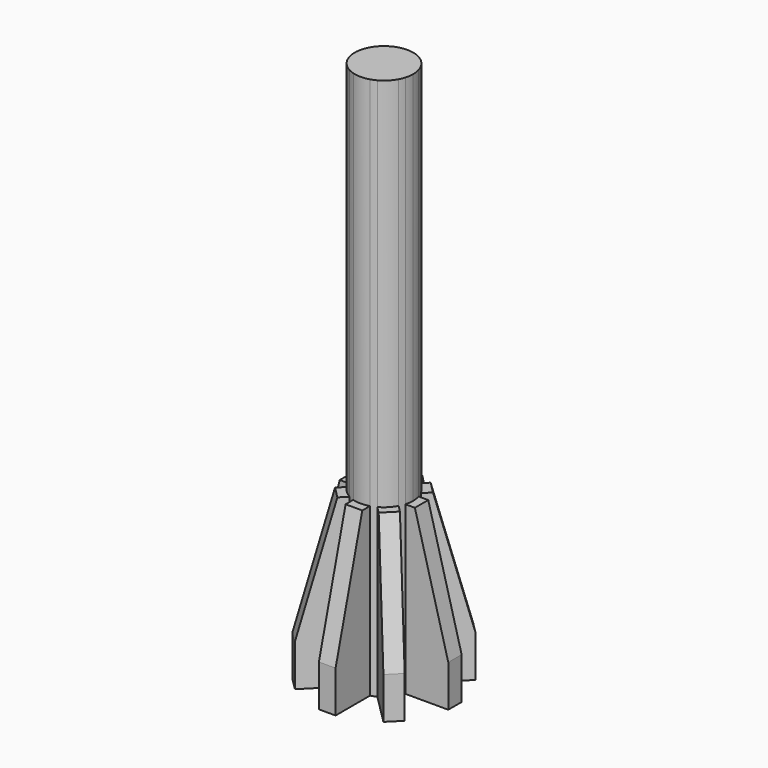
from build123d import *

# Parameters (mm, degrees)
F1_DEPTH   = 65
F2_DEPTH   = 20
F3_SIZE2   = 15
F3_SIZE    = 4
F3_2_SIZE2 = 15
F3_2_SIZE  = 4
F3_3_SIZE2 = 15
F3_3_SIZE  = 4
F3_4_SIZE2 = 15
F3_4_SIZE  = 4
F4_SIZE2   = 4
F4_SIZE    = 15
F4_2_SIZE2 = 4
F4_2_SIZE  = 15
F4_3_SIZE2 = 4
F4_3_SIZE  = 15
F4_4_SIZE2 = 4
F4_4_SIZE  = 15


with BuildPart() as f1:
    # F0 (on Top) → F1 (new body)
    with BuildSketch(Plane.XY):
        with BuildLine():
            Line((0.4761658125, 5.9305784088), (1.1407672764, 6.5951798727))
            ThreePointArc((1.1407672764, 6.5951798727), (0.8155578257, 6.7499432102), (0.4761658125, 6.8704668126))
            Line((0.4761658125, 6.8704668126), (0.4761658125, 5.9305784088))
        make_face()
        with BuildLine():
            Line((-3.6026492139, 1.8517633824), (-2.9380477499, 2.5163648464))
            Line((-2.9380477499, 2.5163648464), (-3.8779361538, 2.5163648464))
            ThreePointArc((-3.8779361538, 2.5163648464), (-3.7574125513, 2.1769728331), (-3.6026492139, 1.8517633824))
        make_face()
        with BuildLine():
            ThreePointArc((2.8302677787, 4.5163648464), (2.7097441763, 4.8557568597), (2.5549808388, 5.1809663103))
            Line((2.5549808388, 5.1809663103), (1.8903793748, 4.5163648464))
            Line((1.8903793748, 4.5163648464), (2.8302677787, 4.5163648464))
        make_face()
        with BuildLine():
            Line((-1.5238341875, 0.1622628801), (-1.5238341875, 1.102151284))
            Line((-1.5238341875, 1.102151284), (-2.1884356515, 0.4375498201))
            ThreePointArc((-2.1884356515, 0.4375498201), (-1.8632262008, 0.2827864826), (-1.5238341875, 0.1622628801))
        make_face()
        with BuildLine():
            ThreePointArc((2.5549808388, 5.1809663103), (1.9510395466, 5.9912385805), (1.1407672764, 6.5951798727))
            Line((1.1407672764, 6.5951798727), (0.4761658125, 5.9305784088))
            Line((0.4761658125, 5.9305784088), (0.4761658125, 4.5163648464))
            Line((0.4761658125, 4.5163648464), (1.8903793748, 4.5163648464))
            Line((1.8903793748, 4.5163648464), (2.5549808388, 5.1809663103))
        make_face()
        Polygon((-0.9380477499, 4.5163648464), (-0.5238341875, 4.9305784088), (-1.5238341875, 5.9305784088), (-1.5238341875, 4.5163648464), align=None)
        with BuildLine():
            Line((-1.5238341875, 2.5163648464), (-2.9380477499, 2.5163648464))
            Line((-2.9380477499, 2.5163648464), (-3.6026492139, 1.8517633824))
            ThreePointArc((-3.6026492139, 1.8517633824), (-2.9987079217, 1.0414911122), (-2.1884356515, 0.4375498201))
            Line((-2.1884356515, 0.4375498201), (-1.5238341875, 1.102151284))
            Line((-1.5238341875, 1.102151284), (-1.5238341875, 2.5163648464))
        make_face()
        Polygon((1.8903793748, 2.5163648464), (0.8903793748, 3.5163648464), (0.4761658125, 3.102151284), (0.4761658125, 2.5163648464), align=None)
        Polygon((-0.1096206252, 4.5163648464), (-0.5238341875, 4.9305784088), (-0.9380477499, 4.5163648464), align=None)
        with BuildLine():
            Line((-1.5238341875, 4.5163648464), (-1.5238341875, 5.9305784088))
            Line((-1.5238341875, 5.9305784088), (-2.1884356515, 6.5951798727))
            ThreePointArc((-2.1884356515, 6.5951798727), (-2.9987079217, 5.9912385805), (-3.6026492139, 5.1809663103))
            Line((-3.6026492139, 5.1809663103), (-2.9380477499, 4.5163648464))
            Line((-2.9380477499, 4.5163648464), (-1.5238341875, 4.5163648464))
        make_face()
        Polygon((0.4761658125, 2.5163648464), (0.4761658125, 3.102151284), (-0.1096206252, 2.5163648464), align=None)
        with BuildLine():
            Line((-2.9380477499, 2.5163648464), (-1.9380477499, 3.5163648464))
            Line((-1.9380477499, 3.5163648464), (-2.9380477499, 4.5163648464))
            Line((-2.9380477499, 4.5163648464), (-3.8779361538, 4.5163648464))
            ThreePointArc((-3.8779361538, 4.5163648464), (-4.0238341875, 3.5163648464), (-3.8779361538, 2.5163648464))
            Line((-3.8779361538, 2.5163648464), (-2.9380477499, 2.5163648464))
        make_face()
        with BuildLine():
            Line((-0.5238341875, 4.9305784088), (0.4761658125, 5.9305784088))
            Line((0.4761658125, 5.9305784088), (0.4761658125, 6.8704668126))
            ThreePointArc((0.4761658125, 6.8704668126), (-0.5238341875, 7.0163648464), (-1.5238341875, 6.8704668126))
            Line((-1.5238341875, 6.8704668126), (-1.5238341875, 5.9305784088))
            Line((-1.5238341875, 5.9305784088), (-0.5238341875, 4.9305784088))
        make_face()
        with BuildLine():
            Line((2.8302677787, 4.5163648464), (1.8903793748, 4.5163648464))
            Line((1.8903793748, 4.5163648464), (0.8903793748, 3.5163648464))
            Line((0.8903793748, 3.5163648464), (1.8903793748, 2.5163648464))
            Line((1.8903793748, 2.5163648464), (2.8302677787, 2.5163648464))
            ThreePointArc((2.8302677787, 2.5163648464), (2.9394992415, 3.0110713089), (2.9761658125, 3.5163648464))
            ThreePointArc((2.9761658125, 3.5163648464), (2.9394992415, 4.0216583839), (2.8302677787, 4.5163648464))
        make_face()
        Polygon((-1.5238341875, 3.102151284), (-1.5238341875, 3.9305784088), (-1.9380477499, 3.5163648464), align=None)
        Polygon((0.4761658125, 4.5163648464), (0.4761658125, 5.9305784088), (-0.5238341875, 4.9305784088), (-0.1096206252, 4.5163648464), align=None)
        Polygon((-1.5238341875, 3.9305784088), (-0.9380477499, 4.5163648464), (-1.5238341875, 4.5163648464), align=None)
        with BuildLine():
            Line((2.5549808388, 1.8517633824), (1.8903793748, 2.5163648464))
            Line((1.8903793748, 2.5163648464), (0.4761658125, 2.5163648464))
            Line((0.4761658125, 2.5163648464), (0.4761658125, 1.102151284))
            Line((0.4761658125, 1.102151284), (1.1407672764, 0.4375498201))
            ThreePointArc((1.1407672764, 0.4375498201), (1.9510395466, 1.0414911122), (2.5549808388, 1.8517633824))
        make_face()
        Polygon((0.8903793748, 3.5163648464), (0.4761658125, 3.9305784088), (0.4761658125, 3.102151284), align=None)
        Polygon((-0.1096206252, 4.5163648464), (-0.9380477499, 4.5163648464), (-1.5238341875, 3.9305784088), (-1.5238341875, 3.102151284), (-0.9380477499, 2.5163648464), (-0.1096206252, 2.5163648464), (0.4761658125, 3.102151284), (0.4761658125, 3.9305784088), align=None)
        with BuildLine():
            Line((2.8302677787, 2.5163648464), (1.8903793748, 2.5163648464))
            Line((1.8903793748, 2.5163648464), (2.5549808388, 1.8517633824))
            ThreePointArc((2.5549808388, 1.8517633824), (2.7097441763, 2.1769728331), (2.8302677787, 2.5163648464))
        make_face()
        Polygon((0.4761658125, 3.9305784088), (0.4761658125, 4.5163648464), (-0.1096206252, 4.5163648464), align=None)
        Polygon((-1.9380477499, 3.5163648464), (-1.5238341875, 3.9305784088), (-1.5238341875, 4.5163648464), (-2.9380477499, 4.5163648464), align=None)
        with BuildLine():
            Line((0.4761658125, 1.102151284), (-0.5238341875, 2.102151284))
            Line((-0.5238341875, 2.102151284), (-1.5238341875, 1.102151284))
            Line((-1.5238341875, 1.102151284), (-1.5238341875, 0.1622628801))
            ThreePointArc((-1.5238341875, 0.1622628801), (-0.5238341875, 0.0163648464), (0.4761658125, 0.1622628801))
            Line((0.4761658125, 0.1622628801), (0.4761658125, 1.102151284))
        make_face()
        with BuildLine():
            Line((-1.5238341875, 5.9305784088), (-1.5238341875, 6.8704668126))
            ThreePointArc((-1.5238341875, 6.8704668126), (-1.8632262008, 6.7499432102), (-2.1884356515, 6.5951798727))
            Line((-2.1884356515, 6.5951798727), (-1.5238341875, 5.9305784088))
        make_face()
        Polygon((-1.5238341875, 3.102151284), (-1.9380477499, 3.5163648464), (-2.9380477499, 2.5163648464), (-1.5238341875, 2.5163648464), align=None)
        with BuildLine():
            Line((-2.9380477499, 4.5163648464), (-3.6026492139, 5.1809663103))
            ThreePointArc((-3.6026492139, 5.1809663103), (-3.7574125513, 4.8557568597), (-3.8779361538, 4.5163648464))
            Line((-3.8779361538, 4.5163648464), (-2.9380477499, 4.5163648464))
        make_face()
        Polygon((-0.9380477499, 2.5163648464), (-1.5238341875, 3.102151284), (-1.5238341875, 2.5163648464), align=None)
        Polygon((-0.5238341875, 2.102151284), (-0.9380477499, 2.5163648464), (-1.5238341875, 2.5163648464), (-1.5238341875, 1.102151284), align=None)
        Polygon((-0.5238341875, 2.102151284), (-0.1096206252, 2.5163648464), (-0.9380477499, 2.5163648464), align=None)
        Polygon((0.4761658125, 2.5163648464), (-0.1096206252, 2.5163648464), (-0.5238341875, 2.102151284), (0.4761658125, 1.102151284), align=None)
        Polygon((1.8903793748, 4.5163648464), (0.4761658125, 4.5163648464), (0.4761658125, 3.9305784088), (0.8903793748, 3.5163648464), align=None)
        with BuildLine():
            Line((1.1407672764, 0.4375498201), (0.4761658125, 1.102151284))
            Line((0.4761658125, 1.102151284), (0.4761658125, 0.1622628801))
            ThreePointArc((0.4761658125, 0.1622628801), (0.8155578257, 0.2827864826), (1.1407672764, 0.4375498201))
        make_face()
    extrude(amount=F1_DEPTH)

    # F0 (on Top) → F2 (join)
    with BuildSketch(Plane.XY):
        with BuildLine():
            Line((6.1936802337, 8.8196657053), (4.7794666714, 10.2338792677))
            Line((4.7794666714, 10.2338792677), (1.1407672764, 6.5951798727))
            ThreePointArc((1.1407672764, 6.5951798727), (1.9510395466, 5.9912385805), (2.5549808388, 5.1809663103))
            Line((2.5549808388, 5.1809663103), (6.1936802337, 8.8196657053))
        make_face()
        with BuildLine():
            ThreePointArc((-3.6026492139, 5.1809663103), (-2.9987079217, 5.9912385805), (-2.1884356515, 6.5951798727))
            Line((-2.1884356515, 6.5951798727), (-5.8271350464, 10.2338792677))
            Line((-5.8271350464, 10.2338792677), (-7.2413486088, 8.8196657053))
            Line((-7.2413486088, 8.8196657053), (-3.6026492139, 5.1809663103))
        make_face()
        with BuildLine():
            ThreePointArc((-2.1884356515, 0.4375498201), (-2.9987079217, 1.0414911122), (-3.6026492139, 1.8517633824))
            Line((-3.6026492139, 1.8517633824), (-7.2413486088, -1.7869360125))
            Line((-7.2413486088, -1.7869360125), (-5.8271350464, -3.2011495749))
            Line((-5.8271350464, -3.2011495749), (-2.1884356515, 0.4375498201))
        make_face()
        with BuildLine():
            ThreePointArc((-3.8779361538, 2.5163648464), (-4.0238341875, 3.5163648464), (-3.8779361538, 4.5163648464))
            Line((-3.8779361538, 4.5163648464), (-9.0238341875, 4.5163648464))
            Line((-9.0238341875, 4.5163648464), (-9.0238341875, 2.5163648464))
            Line((-9.0238341875, 2.5163648464), (-3.8779361538, 2.5163648464))
        make_face()
        with BuildLine():
            Line((0.4761658125, -4.9836351536), (0.4761658125, 0.1622628801))
            ThreePointArc((0.4761658125, 0.1622628801), (-0.5238341875, 0.0163648464), (-1.5238341875, 0.1622628801))
            Line((-1.5238341875, 0.1622628801), (-1.5238341875, -4.9836351536))
            Line((-1.5238341875, -4.9836351536), (0.4761658125, -4.9836351536))
        make_face()
        with BuildLine():
            Line((7.9761658125, 4.5163648464), (2.8302677787, 4.5163648464))
            ThreePointArc((2.8302677787, 4.5163648464), (2.9394992415, 4.0216583839), (2.9761658125, 3.5163648464))
            ThreePointArc((2.9761658125, 3.5163648464), (2.9394992415, 3.0110713089), (2.8302677787, 2.5163648464))
            Line((2.8302677787, 2.5163648464), (7.9761658125, 2.5163648464))
            Line((7.9761658125, 2.5163648464), (7.9761658125, 4.5163648464))
        make_face()
        with BuildLine():
            Line((6.1936802337, -1.7869360125), (2.5549808388, 1.8517633824))
            ThreePointArc((2.5549808388, 1.8517633824), (1.9510395466, 1.0414911122), (1.1407672764, 0.4375498201))
            Line((1.1407672764, 0.4375498201), (4.7794666714, -3.2011495749))
            Line((4.7794666714, -3.2011495749), (6.1936802337, -1.7869360125))
        make_face()
        with BuildLine():
            ThreePointArc((-1.5238341875, 6.8704668126), (-0.5238341875, 7.0163648464), (0.4761658125, 6.8704668126))
            Line((0.4761658125, 6.8704668126), (0.4761658125, 12.0163648464))
            Line((0.4761658125, 12.0163648464), (-1.5238341875, 12.0163648464))
            Line((-1.5238341875, 12.0163648464), (-1.5238341875, 6.8704668126))
        make_face()
    extrude(amount=F2_DEPTH)

    # F3
    f3_edges = [f1.edges().sort_by_distance(p)[0] for p in [
        (-6.534242, 9.526772, 20),
    ]]
    f3_side = f1.faces().sort_by_distance((-4.749295, 7.741826, 20))[0]
    chamfer(f3_edges, length=F3_SIZE, length2=F3_SIZE2, reference=f3_side)

    # F3#2
    f3_2_edges = [f1.edges().sort_by_distance(p)[0] for p in [
        (-6.534242, -2.494043, 20),
    ]]
    f3_2_side = f1.faces().sort_by_distance((-4.749295, -0.709096, 20))[0]
    chamfer(f3_2_edges, length=F3_2_SIZE, length2=F3_2_SIZE2, reference=f3_2_side)

    # F3#3
    f3_3_edges = [f1.edges().sort_by_distance(p)[0] for p in [
        (-0.523834, 12.016365, 20),
    ]]
    f3_3_side = f1.faces().sort_by_distance((-0.523834, 9.492069, 20))[0]
    chamfer(f3_3_edges, length=F3_3_SIZE, length2=F3_3_SIZE2, reference=f3_3_side)

    # F3#4
    f3_4_edges = [f1.edges().sort_by_distance(p)[0] for p in [
        (-9.023834, 3.516365, 20),
    ]]
    f3_4_side = f1.faces().sort_by_distance((-6.499538, 3.516365, 20))[0]
    chamfer(f3_4_edges, length=F3_4_SIZE, length2=F3_4_SIZE2, reference=f3_4_side)

    # F4
    f4_edges = [f1.edges().sort_by_distance(p)[0] for p in [
        (5.486573, -2.494043, 20),
    ]]
    f4_side = f1.faces().sort_by_distance((5.486573, -2.494043, 10))[0]
    chamfer(f4_edges, length=F4_SIZE, length2=F4_SIZE2, reference=f4_side)

    # F4#2
    f4_2_edges = [f1.edges().sort_by_distance(p)[0] for p in [
        (5.486573, 9.526772, 20),
    ]]
    f4_2_side = f1.faces().sort_by_distance((5.486573, 9.526772, 10))[0]
    chamfer(f4_2_edges, length=F4_2_SIZE, length2=F4_2_SIZE2, reference=f4_2_side)

    # F4#3
    f4_3_edges = [f1.edges().sort_by_distance(p)[0] for p in [
        (-0.523834, -4.983635, 20),
    ]]
    f4_3_side = f1.faces().sort_by_distance((-0.523834, -4.983635, 10))[0]
    chamfer(f4_3_edges, length=F4_3_SIZE, length2=F4_3_SIZE2, reference=f4_3_side)

    # F4#4
    f4_4_edges = [f1.edges().sort_by_distance(p)[0] for p in [
        (7.976166, 3.516365, 20),
    ]]
    f4_4_side = f1.faces().sort_by_distance((7.976166, 3.516365, 10))[0]
    chamfer(f4_4_edges, length=F4_4_SIZE, length2=F4_4_SIZE2, reference=f4_4_side)


solid = f1.part
